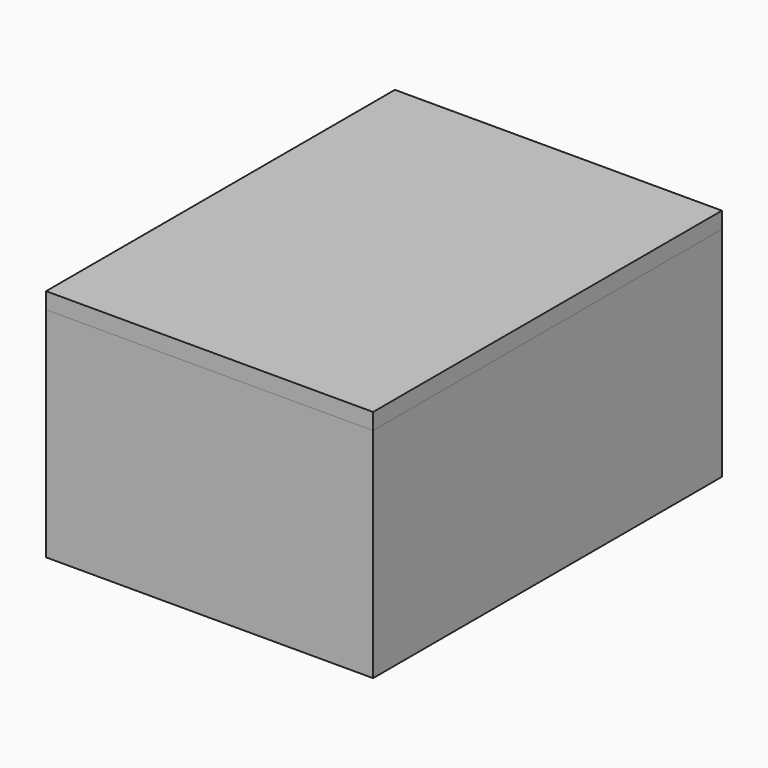
from build123d import *

# Parameters (mm, degrees)
F0_W     = 60
F0_H     = 80
F1_DEPTH = 40
F2_T     = -3
F3_W     = 60
F3_H     = 80
F3_W_2   = 54
F3_H_2   = 74
F4_DEPTH = 3
F5_DEPTH = 4


with BuildPart() as f1:
    # F0 (on Top) → F1 (new body)
    with BuildSketch(Plane.XY):
        Rectangle(F0_W, F0_H)
    extrude(amount=F1_DEPTH)

    # F2
    f2_openings = [f1.faces().sort_by_distance(p)[0] for p in [
        (0, 0, 40),
    ]]
    offset(amount=F2_T, openings=f2_openings)


with BuildPart() as f4:
    # F3 (on face) → F4 (new body)
    with BuildSketch(Plane.XY.offset(40)):
        Rectangle(F3_W, F3_H)
        Rectangle(F3_W_2, F3_H_2, mode=Mode.SUBTRACT)
        Rectangle(F3_W_2, F3_H_2)
    extrude(amount=F4_DEPTH)

    # F3 (on face) → F5 (join)
    with BuildSketch(Plane.XY.offset(40)):
        Rectangle(F3_W_2, F3_H_2)
    extrude(amount=-F5_DEPTH)


solid = Compound([f1.part, f4.part])
